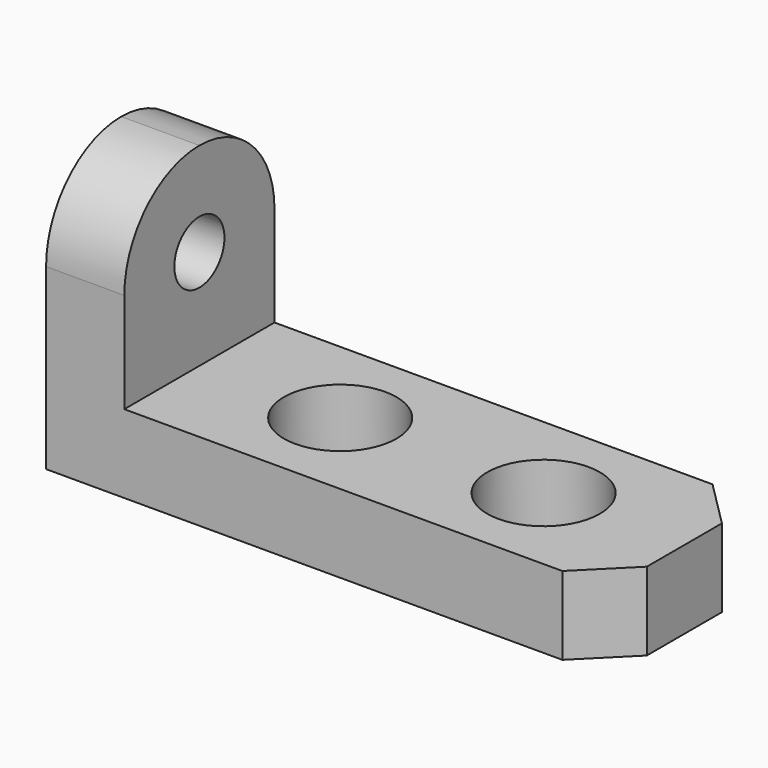
from build123d import *

# Parameters (mm, degrees)
F0_W     = 4572
F0_H     = 1524
F1_DEPTH = 635
F2_W     = 635
F2_H     = 1524
F3_DEPTH = 1574.8
F4_R     = 762
F5_R     = 761.99999
F6_R     = 457.2
F7_DEPTH = 635
F8_R     = 254
F9_DEPTH = 635
F10_SIZE = 381
F11_SIZE = 381


# Not quite as in the source:
# - a fillet or chamfer is up to 0.001 mm smaller than in the source, because OpenCascade refuses the exact size


with BuildPart() as f1:
    # F0 (on Top) → F1 (new body)
    with BuildSketch(Plane.XY):
        with Locations((2286, 762)):
            Rectangle(F0_W, F0_H)
    extrude(amount=F1_DEPTH)

    # F2 (on face) → F3 (join)
    with BuildSketch(Plane.XY.offset(635)):
        with Locations((317.5, 762)):
            Rectangle(F2_W, F2_H)
    extrude(amount=F3_DEPTH)

    # F4
    f4_edges = [f1.edges().sort_by_distance(p)[0] for p in [
        (317.5, 0, 2209.8),
    ]]
    fillet(f4_edges, radius=F4_R)

    # F5 (radius 762 in the source; OpenCascade refuses exactly that, so slightly less here)
    f5_edges = [f1.edges().sort_by_distance(p)[0] for p in [
        (317.5, 1524, 2209.8),
    ]]
    fillet(f5_edges, radius=F5_R)

    # F6 (on face) → F7 (cut, through all)
    with BuildSketch(Plane.XY.offset(635)):
        with Locations((1778, 762)):
            Circle(F6_R)
        with Locations((3429, 762)):
            Circle(F6_R)
    extrude(amount=-F7_DEPTH, mode=Mode.SUBTRACT)

    # F8 (on face) → F9 (cut, through all)
    with BuildSketch(Plane.YZ.offset(635)):
        with Locations((762, 1447.8)):
            Circle(F8_R)
    extrude(amount=-F9_DEPTH, mode=Mode.SUBTRACT)

    # F10
    f10_edges = [f1.edges().sort_by_distance(p)[0] for p in [
        (4572, 0, 317.5),
    ]]
    chamfer(f10_edges, length=F10_SIZE)

    # F11
    f11_edges = [f1.edges().sort_by_distance(p)[0] for p in [
        (4572, 1524, 317.5),
    ]]
    chamfer(f11_edges, length=F11_SIZE)


solid = f1.part
